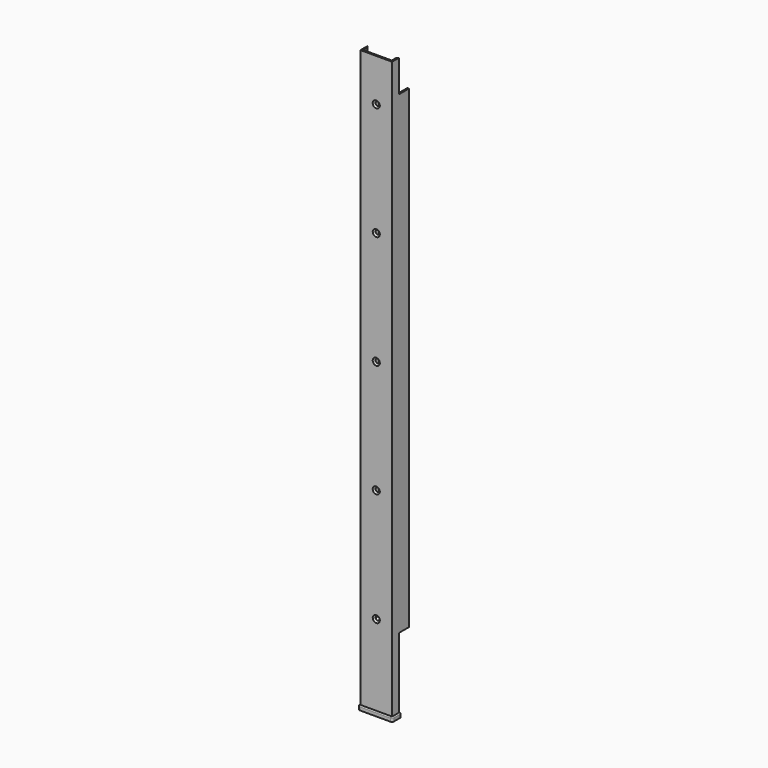
from build123d import *

# Parameters (mm, degrees)
F1_DEPTH        = 1100
F7_R            = 40
F8_DEPTH        = 139
F10_R           = 40
F11_DEPTH       = 61
F13_D           = 6.6
F13_CSINK_D     = 13.44
F13_CSINK_ANGLE = 90
F15_DEPTH       = 6
F16_DEPTH       = 2
F17_R           = 3.9
F18_T1_DEPTH    = 13.9424868894
F18_T3_DEPTH    = 11
F18_T5_DEPTH    = 0.4
F18_T7_DEPTH    = 57.4
F18_T9_DEPTH    = 5.7424868894
F18_T11_DEPTH   = 41
F18_T13_DEPTH   = 0.4
F18_T16_ANGLE   = 90
F18_T18_ANGLE   = 90
F18_T20_ANGLE   = 90
F18_T22_ANGLE   = 90
F18_T24_ANGLE   = 90
F18_T26_ANGLE   = 90
F18_T28_ANGLE   = 90
F18_T30_ANGLE   = 90


# Not quite as in the source:
# - a fillet or chamfer that OpenCascade refuses, or shapes differently, is made with other operations: its cross-section is extruded or revolved along the edge and cut away or added


with BuildPart() as f1:
    # F0 (on Top) → F1 (new body)
    with BuildSketch(Plane.XY):
        Polygon((-60, 0), (0, 0), (0, 40), (-3, 40), (-3, 3), (-57, 3), (-57, 40), (-60, 40), align=None)
    extrude(amount=F1_DEPTH)

    # F7 (on offset) → F8 (cut, through all)
    with BuildSketch(Plane.XY.offset(139)):
        with Locations((-30, 43)):
            Circle(F7_R)
    extrude(amount=-F8_DEPTH, mode=Mode.SUBTRACT)

    # F10 (on offset) → F11 (cut, through all)
    with BuildSketch(Plane.XY.offset(1039)):
        with Locations((-30, 43)):
            Circle(F10_R)
    extrude(amount=F11_DEPTH, mode=Mode.SUBTRACT)

    # F13 (through all)
    with Locations(Plane.XZ):
        with Locations((-30, 159), (-30, 374), (-30, 589), (-30, 804), (-30, 1019)):
            CounterSinkHole(F13_D / 2, F13_CSINK_D / 2, counter_sink_angle=F13_CSINK_ANGLE)


with BuildPart() as f15:
    # F14 (on face) → F15 (new body)
    with BuildSketch(Plane(origin=(0, 0, 0), x_dir=(1, 0, 0), z_dir=(0, 0, -1))):
        Polygon((2.6, -19.1424868894), (2.6, 2.6), (-62.6, 2.6), (-62.6, -19.1424868894), (-54.4, -19.1424868894), (-54.4, -5.6), (-5.6, -5.6), (-5.6, -19.1424868894), align=None)
        Polygon((-60.2, 0.2), (0.2, 0.2), (0.2, -16.7424868894), (-3.2, -16.7424868894), (-3.2, -3.2), (-56.8, -3.2), (-56.8, -16.7424868894), (-60.2, -16.7424868894), align=None, mode=Mode.SUBTRACT)
    extrude(amount=-F15_DEPTH)

    # F14 (on face) → F16 (join)
    with BuildSketch(Plane(origin=(0, 0, 0), x_dir=(1, 0, 0), z_dir=(0, 0, -1))):
        Polygon((2.6, -19.1424868894), (2.6, 2.6), (-62.6, 2.6), (-62.6, -19.1424868894), (-54.4, -19.1424868894), (-54.4, -5.6), (-5.6, -5.6), (-5.6, -19.1424868894), align=None)
        Polygon((-60.2, 0.2), (0.2, 0.2), (0.2, -16.7424868894), (-3.2, -16.7424868894), (-3.2, -3.2), (-56.8, -3.2), (-56.8, -16.7424868894), (-60.2, -16.7424868894), align=None, mode=Mode.SUBTRACT)
        Polygon((0.2, -16.7424868894), (0.2, 0.2), (-60.2, 0.2), (-60.2, -16.7424868894), (-56.8, -16.7424868894), (-56.8, -3.2), (-3.2, -3.2), (-3.2, -16.7424868894), align=None)
        with BuildLine():
            Line((-60, -16.5424868894), (-60, 0))
            Line((-60, 0), (0, 0))
            Line((0, 0), (0, -16.5424868894))
            ThreePointArc((0, -16.5424868894), (-1.459089789, -14.9747177655), (-3, -13.4872908733))
            Line((-3, -13.4872908733), (-3, -3))
            Line((-3, -3), (-30, -3))
            Line((-30, -3), (-57, -3))
            Line((-57, -3), (-57, -13.4872908733))
            ThreePointArc((-57, -13.4872908733), (-58.540910211, -14.9747177655), (-60, -16.5424868894))
        make_face(mode=Mode.SUBTRACT)
        with BuildLine():
            Line((0, 0), (-60, 0))
            Line((-60, 0), (-60, -16.5424868894))
            ThreePointArc((-60, -16.5424868894), (-58.540910211, -14.9747177655), (-57, -13.4872908733))
            Line((-57, -13.4872908733), (-57, -3))
            Line((-57, -3), (-30, -3))
            Line((-30, -3), (-3, -3))
            Line((-3, -3), (-3, -13.4872908733))
            ThreePointArc((-3, -13.4872908733), (-1.459089789, -14.9747177655), (0, -16.5424868894))
            Line((0, -16.5424868894), (0, 0))
        make_face()
    extrude(amount=F16_DEPTH)

    # F17
    f17_edges = [f15.edges().sort_by_distance(p)[0] for p in [
        (2.6, 19.142487, 2),
        (-5.6, 19.142487, 2),
        (-5.6, 5.6, 2),
        (-54.4, 19.142487, 2),
        (-62.6, 19.142487, 2),
        (-54.4, 5.6, 2),
        (-62.6, -2.6, 2),
        (2.6, -2.6, 2),
    ]]
    fillet(f17_edges, radius=F17_R)

    # F18: fillet of radius 2 on 18 edges, made by hand

    # F18_s2 → F18_t1 (cut)
    with BuildSketch(Plane.XZ.offset(-15.2424868894)):
        with BuildLine():
            ThreePointArc((2.6, 4), (2.0142135624, 5.4142135624), (0.6, 6))
            Line((0.6, 6), (2.6, 6))
            Line((2.6, 6), (2.6, 4))
        make_face()
        with BuildLine():
            ThreePointArc((-60.6, 6), (-62.0142135624, 5.4142135624), (-62.6, 4))
            Line((-62.6, 4), (-62.6, 6))
            Line((-62.6, 6), (-60.6, 6))
        make_face()
    extrude(amount=F18_T1_DEPTH, mode=Mode.SUBTRACT)

    # F18_s4 → F18_t3 (cut)
    with BuildSketch(Plane.XY):
        with BuildLine():
            ThreePointArc((-3.2, 5.2), (-3.7857864376, 3.7857864376), (-5.2, 3.2))
            Line((-5.2, 3.2), (-3.2, 3.2))
            Line((-3.2, 3.2), (-3.2, 5.2))
        make_face()
        with BuildLine():
            ThreePointArc((-54.8, 3.2), (-56.2142135624, 3.7857864376), (-56.8, 5.2))
            Line((-56.8, 5.2), (-56.8, 3.2))
            Line((-56.8, 3.2), (-54.8, 3.2))
        make_face()
    extrude(amount=F18_T3_DEPTH, mode=Mode.SUBTRACT)

    # F18_s6 → F18_t5 (cut)
    with BuildSketch(Plane.YZ.offset(-1.7)):
        with BuildLine():
            ThreePointArc((17.1424868894, 6), (18.5567004517, 5.4142135624), (19.1424868894, 4))
            Line((19.1424868894, 4), (19.1424868894, 6))
            Line((19.1424868894, 6), (17.1424868894, 6))
        make_face()
    extrude(amount=F18_T5_DEPTH, mode=Mode.SUBTRACT)

    # F18_s8 → F18_t7 (cut)
    with BuildSketch(Plane.YZ.offset(-58.7)):
        with BuildLine():
            ThreePointArc((-0.6, 6), (-2.0142135624, 5.4142135624), (-2.6, 4))
            Line((-2.6, 4), (-2.6, 6))
            Line((-2.6, 6), (-0.6, 6))
        make_face()
    extrude(amount=F18_T7_DEPTH, mode=Mode.SUBTRACT)

    # F18_s10 → F18_t9 (cut)
    with BuildSketch(Plane.XZ.offset(-15.2424868894)):
        with BuildLine():
            ThreePointArc((-3.6, 6), (-5.0142135624, 5.4142135624), (-5.6, 4))
            Line((-5.6, 4), (-5.6, 6))
            Line((-5.6, 6), (-3.6, 6))
        make_face()
        with BuildLine():
            ThreePointArc((-56.4, 6), (-54.9857864376, 5.4142135624), (-54.4, 4))
            Line((-54.4, 4), (-54.4, 6))
            Line((-54.4, 6), (-56.4, 6))
        make_face()
    extrude(amount=F18_T9_DEPTH, mode=Mode.SUBTRACT)

    # F18_s12 → F18_t11 (cut)
    with BuildSketch(Plane.YZ.offset(-50.5)):
        with BuildLine():
            ThreePointArc((3.6, 6), (5.0142135624, 5.4142135624), (5.6, 4))
            Line((5.6, 4), (5.6, 6))
            Line((5.6, 6), (3.6, 6))
        make_face()
    extrude(amount=F18_T11_DEPTH, mode=Mode.SUBTRACT)

    # F18_s14 → F18_t13 (cut)
    with BuildSketch(Plane.YZ.offset(-58.7)):
        with BuildLine():
            ThreePointArc((17.1424868894, 6), (18.5567004517, 5.4142135624), (19.1424868894, 4))
            Line((19.1424868894, 4), (19.1424868894, 6))
            Line((19.1424868894, 6), (17.1424868894, 6))
        make_face()
    extrude(amount=F18_T13_DEPTH, mode=Mode.SUBTRACT)

    # F18_s15 → F18_t16 (revolve, cut)
    with BuildSketch(Plane.XZ.offset(-15.2424868894)):
        with BuildLine():
            ThreePointArc((0.6, 6), (2.0142135624, 5.4142135624), (2.6, 4))
            Line((2.6, 4), (2.6, 6))
            Line((2.6, 6), (0.6, 6))
        make_face()
    revolve(axis=Axis((-1.3, 15.2424868894, 6), (0, 0, 1)), revolution_arc=F18_T16_ANGLE, mode=Mode.SUBTRACT)

    # F18_s17 → F18_t18 (revolve, cut)
    with BuildSketch(Plane.XZ.offset(-1.3)):
        with BuildLine():
            ThreePointArc((0.6, 6), (2.0142135624, 5.4142135624), (2.6, 4))
            Line((2.6, 4), (2.6, 6))
            Line((2.6, 6), (0.6, 6))
        make_face()
    revolve(axis=Axis((-1.3, 1.3, 6), (0, 0, -1)), revolution_arc=F18_T18_ANGLE, mode=Mode.SUBTRACT)

    # F18_s19 → F18_t20 (revolve, cut)
    with BuildSketch(Plane.YZ.offset(-1.7)):
        with BuildLine():
            ThreePointArc((17.1424868894, 6), (18.5567004517, 5.4142135624), (19.1424868894, 4))
            Line((19.1424868894, 4), (19.1424868894, 6))
            Line((19.1424868894, 6), (17.1424868894, 6))
        make_face()
    revolve(axis=Axis((-1.7, 15.2424868894, 6), (0, 0, 1)), revolution_arc=F18_T20_ANGLE, mode=Mode.SUBTRACT)

    # F18_s21 → F18_t22 (revolve, cut)
    with BuildSketch(Plane.XZ.offset(-1.3)):
        with BuildLine():
            ThreePointArc((-60.6, 6), (-62.0142135624, 5.4142135624), (-62.6, 4))
            Line((-62.6, 4), (-62.6, 6))
            Line((-62.6, 6), (-60.6, 6))
        make_face()
    revolve(axis=Axis((-58.7, 1.3, 6), (0, 0, 1)), revolution_arc=F18_T22_ANGLE, mode=Mode.SUBTRACT)

    # F18_s23 → F18_t24 (revolve, cut)
    with BuildSketch(Plane.XZ.offset(-9.5)):
        with BuildLine():
            ThreePointArc((-3.6, 6), (-5.0142135624, 5.4142135624), (-5.6, 4))
            Line((-5.6, 4), (-5.6, 6))
            Line((-5.6, 6), (-3.6, 6))
        make_face()
    revolve(axis=Axis((-9.5, 9.5, 6), (0, 0, -1)), revolution_arc=F18_T24_ANGLE, mode=Mode.SUBTRACT)

    # F18_s25 → F18_t26 (revolve, cut)
    with BuildSketch(Plane.YZ.offset(-58.7)):
        with BuildLine():
            ThreePointArc((17.1424868894, 6), (18.5567004517, 5.4142135624), (19.1424868894, 4))
            Line((19.1424868894, 4), (19.1424868894, 6))
            Line((19.1424868894, 6), (17.1424868894, 6))
        make_face()
    revolve(axis=Axis((-58.7, 15.2424868894, 6), (0, 0, 1)), revolution_arc=F18_T26_ANGLE, mode=Mode.SUBTRACT)

    # F18_s27 → F18_t28 (revolve, cut)
    with BuildSketch(Plane.YZ.offset(-50.5)):
        with BuildLine():
            ThreePointArc((3.6, 6), (5.0142135624, 5.4142135624), (5.6, 4))
            Line((5.6, 4), (5.6, 6))
            Line((5.6, 6), (3.6, 6))
        make_face()
    revolve(axis=Axis((-50.5, 9.5, 6), (0, 0, -1)), revolution_arc=F18_T28_ANGLE, mode=Mode.SUBTRACT)

    # F18_s29 → F18_t30 (revolve, cut)
    with BuildSketch(Plane.XZ.offset(-15.2424868894)):
        with BuildLine():
            ThreePointArc((-56.4, 6), (-54.9857864376, 5.4142135624), (-54.4, 4))
            Line((-54.4, 4), (-54.4, 6))
            Line((-54.4, 6), (-56.4, 6))
        make_face()
    revolve(axis=Axis((-58.3, 15.2424868894, 6), (0, 0, 1)), revolution_arc=F18_T30_ANGLE, mode=Mode.SUBTRACT)


solid = Compound([f1.part, f15.part])
